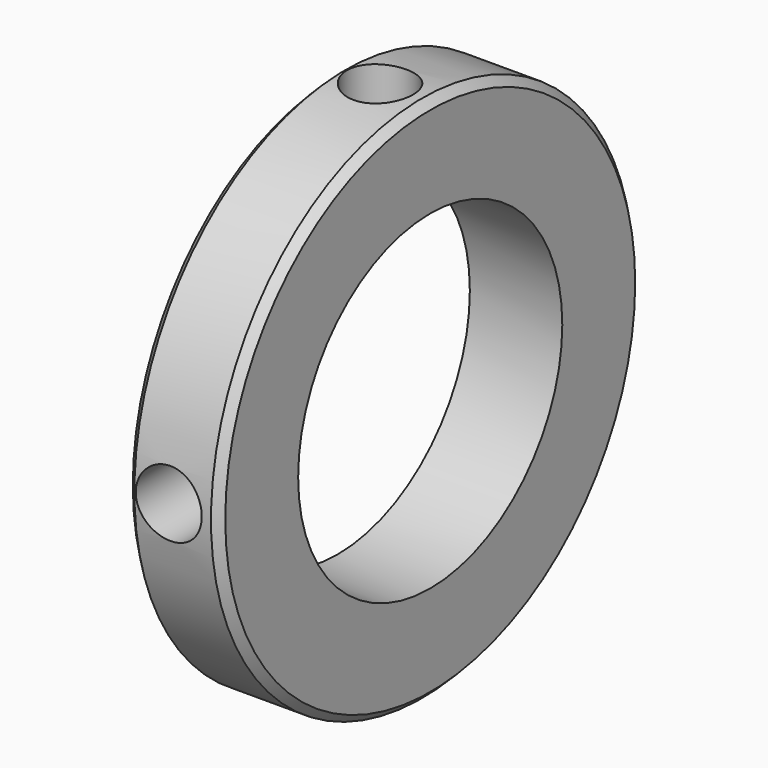
from build123d import *

# Parameters (mm, degrees)
F0_R     = 25.4
F0_R_2   = 15.875
F1_DEPTH = 8.89
F3_R     = 3.175
F4_REACH = 59.7812561211
F6_R     = 3.175
F7_REACH = 59.7812562211
F8_SIZE  = 0.762
F9_SIZE  = 0.762


with BuildPart() as f1:
    # F0 (on Right) → F1 (new body)
    with BuildSketch(Plane.YZ):
        Circle(F0_R)
        Circle(F0_R_2, mode=Mode.SUBTRACT)
    extrude(amount=F1_DEPTH)

    f4_end = f1.faces().sort_by_distance((4.445, -15.875, 0))[0]
    # F3 (on offset) → F4 (cut, up to a face of the model that its end follows)
    with BuildSketch(Plane.XZ.offset(25.4)):
        with Locations((4.064, 0)):
            Circle(F3_R)
    f4_long = extrude(amount=-F4_REACH, mode=Mode.PRIVATE)
    add(split(f4_long, bisect_by=f4_end, keep=Keep.ALL, mode=Mode.PRIVATE).solids().sort_by_distance((4.064, -25.4, 0))[0], mode=Mode.SUBTRACT)

    f7_end = f1.faces().sort_by_distance((0.457728864, -15.875, 0))[0]
    # F6 (on offset) → F7 (cut, up to a face of the model that its end follows)
    with BuildSketch(Plane.XY.offset(25.4)):
        with Locations((4.064, 0)):
            Circle(F6_R)
    f7_long = extrude(amount=-F7_REACH, mode=Mode.PRIVATE)
    add(split(f7_long, bisect_by=f7_end, keep=Keep.ALL, mode=Mode.PRIVATE).solids().sort_by_distance((4.064, 0, 25.4))[0], mode=Mode.SUBTRACT)

    # F8
    f8_edges = [f1.edges().sort_by_distance(p)[0] for p in [
        (0, -25.4, 0),
    ]]
    chamfer(f8_edges, length=F8_SIZE)

    # F9
    f9_edges = [f1.edges().sort_by_distance(p)[0] for p in [
        (8.89, -25.4, 0),
    ]]
    chamfer(f9_edges, length=F9_SIZE)


solid = f1.part
